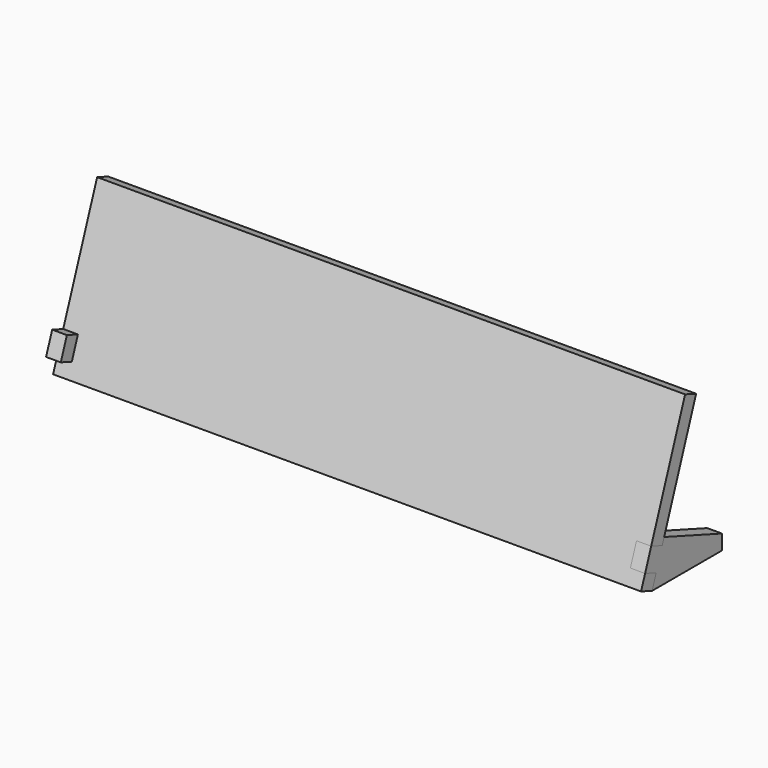
from build123d import *

# Parameters (mm, degrees)
F0_W     = 6.35
F0_H     = 44.45
F1_DEPTH = 20
F3_DEPTH = 6.35
F6_DEPTH = 6.35
F7_DEPTH = 6.35


# Not quite as in the source:
# - a feature names something its author has since deleted; it is built from what else it names


with BuildPart() as f1:
    # F0 (on Top) → F1 (new body)
    with BuildSketch(Plane.XY):
        with Locations((-123.825, 22.225)):
            Rectangle(F0_W, F0_H)
    extrude(amount=F1_DEPTH)

    # F2 (on face) → F3 (cut, through all)
    with BuildSketch(Plane(origin=(-127, 0, 0), x_dir=(0, -1, 0), z_dir=(-1, 0, 0))):
        Polygon((-13.2464528273, 17.8281720899), (-7.2794046853, 20), (-14.0369335405, 20), align=None)
        Polygon((0, 20), (-7.2794046853, 20), (-6.2533442553, 17.1809221376), (-2.9623086233, 8.1388760521), (-0.7904807132, 2.1718279101), (-6.7575288552, 0), (0, 0), align=None)
        Polygon((-44.45, 17.8281720899), (-13.2464528273, 17.8281720899), (-14.0369335405, 20), (-44.45, 20), align=None)
        Polygon((-44.45, 6.4710097155), (-13.2464528273, 17.8281720899), (-44.45, 17.8281720899), align=None)
        Polygon((-6.2533442553, 17.1809221376), (-7.2794046853, 20), (-13.2464528273, 17.8281720899), (-12.2203923973, 15.0090942275), align=None)
        Polygon((-0.7904807132, 2.1718279101), (-2.9623086233, 8.1388760521), (-8.9293567653, 5.967048142), (-6.7575288552, 0), align=None)
    extrude(amount=-F3_DEPTH, mode=Mode.SUBTRACT)


with BuildPart() as f4_1:
    # F4: instance of F1
    add(f1.part.mirror(Plane.YZ))


with BuildPart() as f6:
    # F5 (on face) → F6 (new body)
    with BuildSketch(Plane(origin=(0, 0, 0), x_dir=(1, 0, 0), z_dir=(0, -0.9396926208, 0.3420201433))):
        Polygon((127, 8.6612109876), (120.65, 8.6612109876), (120.65, 18.2835554495), (127, 18.2835554495), (127, 71.8112109876), (-127, 71.8112109876), (-127, 18.2835554495), (-120.65, 18.2835554495), (-120.65, 8.6612109876), (-127, 8.6612109876), (-127, 2.3112109876), (127, 2.3112109876), align=None)
    extrude(amount=-F6_DEPTH)


with BuildPart() as f7:
    # F7 (new): a face of the model
    f7_faces = [f1.part.faces().sort_by_distance(p)[0] for p in [
        (-123.825, 4.6078264393, 12.6598990949),
    ]]
    extrude(f7_faces, amount=F7_DEPTH)


solid = Compound([f1.part, f4_1.part, f6.part, f7.part])
